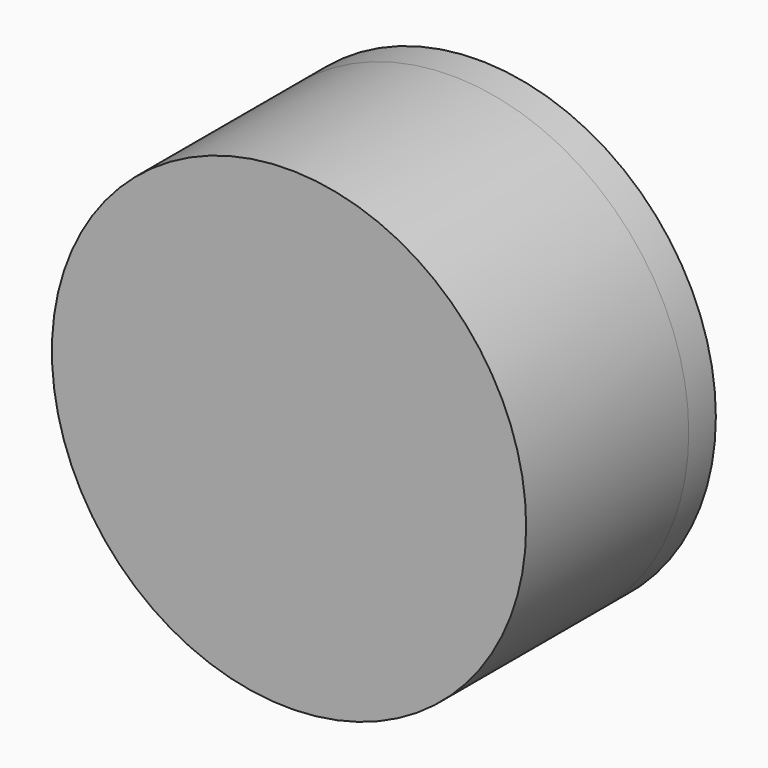
from build123d import *

# Parameters (mm, degrees)
F2_R     = 52.07
F3_DEPTH = 50.8
F2_R_2   = 53.34
F0_DEPTH = 7.62
F1_DEPTH = 43.18
F4_T     = -2.54
F5_R     = 53.34
F6_DEPTH = 2.54


with BuildPart() as f3:
    # F2 (on Front) → F3 (new body)
    with BuildSketch(Plane.XZ):
        Circle(F2_R)
    extrude(amount=F3_DEPTH)

    # F2 (on Front) → F0 (join)
    with BuildSketch(Plane.XZ):
        Circle(F2_R_2)
        Circle(F2_R, mode=Mode.SUBTRACT)
    extrude(amount=F0_DEPTH)


with BuildPart() as f1:
    # F1 (new): a face of the model
    f1_faces = [f3.part.faces().sort_by_distance(p)[0] for p in [
        (-53.1891316972, -7.62, 0),
    ]]
    extrude(f1_faces, amount=F1_DEPTH)

    # F5 (on face) → F6 (join)
    with BuildSketch(Plane.XZ.offset(50.8)):
        Circle(F5_R)
    extrude(amount=F6_DEPTH)


with BuildPart() as f3_1:
    add(f3.part)

    # F4
    f4_openings = [f3_1.faces().sort_by_distance(p)[0] for p in [
        (0, -50.8, 0),
    ]]
    offset(amount=F4_T, openings=f4_openings, kind=Kind.INTERSECTION)


solid = Compound([f1.part, f3_1.part])
